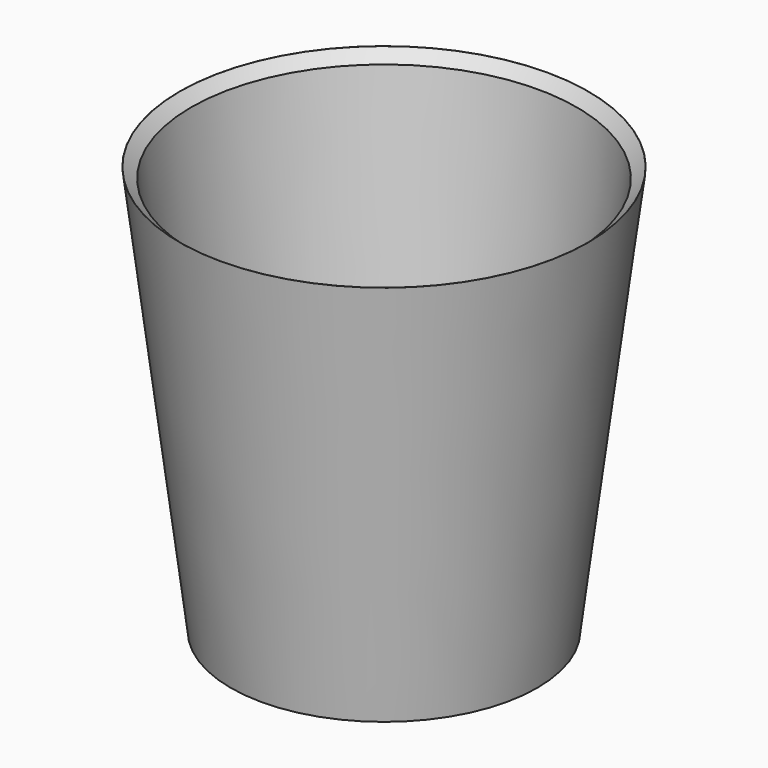
from build123d import *

# Parameters (mm, degrees)
F2_R     = 50.8
F0_R     = 38.1
F4_T     = -2.54
F5_W     = 12.7
F5_H     = 6.35
F6_DEPTH = 40.132
F8_R     = 19.05
F9_DEPTH = 25.4


# Not quite as in the source:
# - a fillet or chamfer that OpenCascade refuses, or shapes differently, is made with other operations: its cross-section is extruded or revolved along the edge and cut away or added


with BuildPart() as f3:
    # F2 (on offset) → F3 section 0
    with BuildSketch(Plane.XY.offset(101.6)):
        Circle(F2_R)
    # F0 (on Top) → F3 section 1
    with BuildSketch(Plane.XY):
        Circle(F0_R)
    loft()

    # F4
    f4_openings = [f3.faces().sort_by_distance(p)[0] for p in [
        (0, 0, 101.6),
    ]]
    offset(amount=F4_T, openings=f4_openings, kind=Kind.INTERSECTION)

    # F5 (on Front) → F6 (cut)
    with BuildSketch(Plane.XZ):
        with Locations((0, 6.35)):
            Rectangle(F5_W, F5_H)
    extrude(amount=-F6_DEPTH, mode=Mode.SUBTRACT)

    # F7: chamfer of 2.54 on 1 edges, made by hand

    # F7_s1 → F7_t2 (revolve, cut)
    with BuildSketch(Plane.XZ):
        Polygon((50.7802331649, 101.6), (47.9251849391, 99.0796141931), (48.2402331649, 101.6), align=None)
    revolve(axis=Axis((0, 0, 101.6), (0, 0, -1)), mode=Mode.SUBTRACT)

    # F8 (on face) → F9 (cut)
    with BuildSketch(Plane.XY.offset(2.54)):
        Circle(F8_R)
    extrude(amount=-F9_DEPTH, mode=Mode.SUBTRACT)


solid = f3.part
